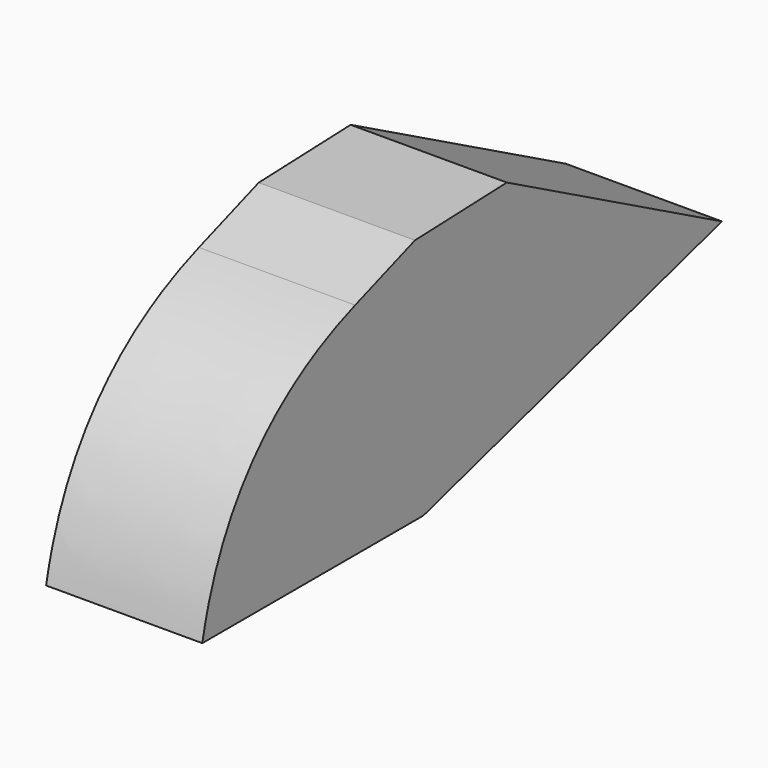
from build123d import *

# Parameters (mm, degrees)
F1_DEPTH    = 25.4
F2_T1_DEPTH = 238.6235911332
F3_SIZE2    = 7.62
F3_SIZE     = 12.7


# Not quite as in the source:
# - a fillet or chamfer that OpenCascade refuses, or shapes differently, is made with other operations: its cross-section is extruded or revolved along the edge and cut away or added


with BuildPart() as f1:
    # F0 (on Right) → F1 (new body)
    with BuildSketch(Plane.YZ):
        Polygon((-44.9345260859, 0), (0, 0), (60.6710910797, 17.4429379404), (10.2382460609, 44.3657338619), (-54.0351904929, 21.4244797826), align=None)
    extrude(amount=F1_DEPTH)

    # F2: fillet of radius 48.2774474346 on 1 edges, made by hand

    # F2_s2 → F2_t1 (cut)
    with BuildSketch(Plane.YZ.offset(-106.6117955666)):
        with BuildLine():
            add(Edge.make_bspline(
                [(-44.9345260859, 0), (-39.4692303476, 26.6235388421), (-13.8721919012, 35.7599440845)],
                knots=[0, 0, 0, 1, 1, 1], degree=2, weights=[1, 1, 1]))
            Line((-13.8721919012, 35.7599440845), (-54.0351904929, 21.4244797826))
            Line((-54.0351904929, 21.4244797826), (-44.9345260859, 0))
        make_face()
    extrude(amount=F2_T1_DEPTH, mode=Mode.SUBTRACT)

    # F3
    f3_edges = [f1.edges().sort_by_distance(p)[0] for p in [
        (12.7, 10.238246, 44.365734),
    ]]
    f3_side = f1.faces().sort_by_distance((12.7, -1.816973, 40.062839))[0]
    chamfer(f3_edges, length=F3_SIZE, length2=F3_SIZE2, reference=f3_side)


solid = f1.part
